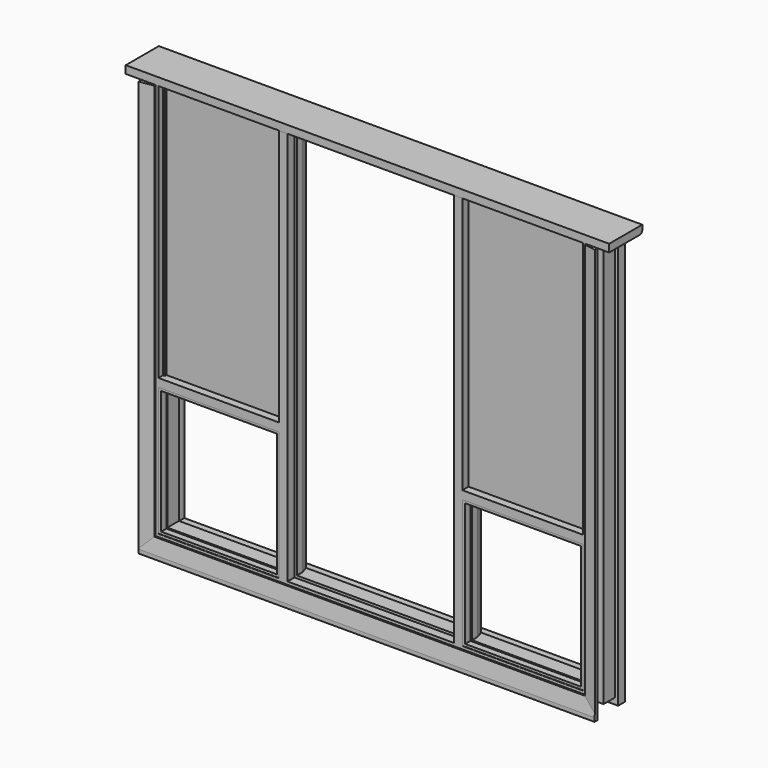
from build123d import *

# Parameters (mm, degrees)
F0_W          = 625
F0_H          = 667
F1_DEPTH      = 45
F3_W          = 645
F3_H          = 687
F3_W_2        = 599
F3_H_2        = 641
F4_DEPTH      = 34
F7_DEPTH      = 75
F9_DEPTH      = 20
F10_T1_DEPTH  = 2228
F10_T3_DEPTH  = 2249.90940659
F10_T9_DEPTH  = 2249.90940659
F10_T15_DEPTH = 2422.90940659
F10_T23_DEPTH = 2422.90940659
F10_T28_DEPTH = 2249.90940659
F11_SIZE2     = 40
F11_SIZE      = 12.5
F13_DEPTH     = 10
F15_DEPTH     = 620
F16_W         = 45
F16_H         = 1126
F17_DEPTH     = 15
F18_T4_DEPTH  = 1160.9259151598
F18_T10_DEPTH = 1160.9259151598
F18_T16_DEPTH = 1160.9259151598
F18_T22_DEPTH = 1160.9259151598
F20_DEPTH     = 44
F22_DEPTH     = 40
F23_R         = 15


# Not quite as in the source:
# - a fillet or chamfer that OpenCascade refuses, or shapes differently, is made with other operations: its cross-section is extruded or revolved along the edge and cut away or added
# - a pattern or mirror of a feature is missing from the dataset's text; its kind, count and spacing are read off the source's solid


with BuildPart() as f1:
    # F0 (on Front) → F1 (new body)
    with BuildSketch(Plane.XZ):
        Polygon((474, 0), (431, 0), (431, -2040), (-431, -2040), (-431, 0), (-474, 0), (-474, -1330), (-1099, -1330), (-1099, 0), (-1124, 0), (-1124, -2065), (1124, -2065), (1124, 0), (1099, 0), (1099, -1330), (474, -1330), align=None)
        with Locations((-786.5, -1706.5)):
            Rectangle(F0_W, F0_H, mode=Mode.SUBTRACT)
        with Locations((786.5, -1706.5)):
            Rectangle(F0_W, F0_H, mode=Mode.SUBTRACT)
    extrude(amount=F1_DEPTH)

    # F3 (on offset) → F4 (join)
    with BuildSketch(Plane.XZ.offset(43)):
        with Locations((786.5, -1706.5)):
            Rectangle(F3_W, F3_H)
        with Locations((786.5, -1706.5)):
            Rectangle(F3_W_2, F3_H_2, mode=Mode.SUBTRACT)
    extrude(amount=-F4_DEPTH)

    # F6: F1 across plane


with BuildPart() as f1_1:
    add(f1.part)
    add(f1.part.mirror(Plane.YZ))

    # F5 (on face) → F7 (join)
    with BuildSketch(Plane(origin=(0, 0, 0), x_dir=(-1, 0, 0), z_dir=(0, 1, 0))):
        Polygon((-488, -2027), (-1099, -2027), (-1099, 0), (-1169, 0), (-1169, -2097), (1169, -2097), (1169, 0), (1099, 0), (1099, -2027), (488, -2027), (488, 0), (418, 0), (418, -2027), (-418, -2027), (-418, 0), (-488, 0), align=None)
    extrude(amount=F7_DEPTH)

    # F8 (on face) → F9 (join)
    with BuildSketch(Plane.XZ.offset(45)):
        Polygon((1114, 0), (1114, -2055), (-1114, -2055), (-1114, 0), (-1187, 0), (-1187, -2150), (1174, -2150), (1174, 0), align=None)
    extrude(amount=F9_DEPTH)

    # F10: chamfer of 12 x 75 on 3 edges, made by hand

    # F10_s2 → F10_t1 (cut)
    with BuildSketch(Plane.YZ.offset(-1114)):
        Polygon((-53, -2055), (-65, -2130), (-65, -2055), align=None)
    extrude(amount=F10_T1_DEPTH, mode=Mode.SUBTRACT)

    # F10_s4 → F10_t3 (cut)
    with BuildSketch(Plane.XY.offset(-2055)):
        Polygon((-1114, -53), (-1189, -65), (-1114, -65), align=None)
        Polygon((1114, -53), (1189, -65), (1114, -65), align=None)
    extrude(amount=F10_T3_DEPTH, mode=Mode.SUBTRACT)


with BuildPart() as f10_tool7:
    # F10_s8 → F10_t9 (new body)
    with BuildSketch(Plane.XY):
        Polygon((1114, -53), (1189, -65), (1114, -65), align=None)
    extrude(amount=-F10_T9_DEPTH)

    split(bisect_by=Plane.XY.offset(-2055), keep=Keep.BOTTOM)

    split(bisect_by=Plane.YZ.offset(1174), keep=Keep.BOTTOM)

    split(bisect_by=Plane.XY.offset(-2150), keep=Keep.TOP)


with BuildPart() as f10_tool13:
    # F10_s14 → F10_t15 (new body)
    with BuildSketch(Plane.YZ.offset(1308.90940659)):
        Polygon((-53, -2055), (-65, -2130), (-65, -2055), align=None)
    extrude(amount=-F10_T15_DEPTH)

    split(bisect_by=Plane.YZ.offset(1114), keep=Keep.TOP)

    split(bisect_by=Plane.YZ.offset(1174), keep=Keep.BOTTOM)


with BuildPart() as f10_tool7_1:
    add(f10_tool7.part)

    # F10_t18: intersect F10_tool13
    add(f10_tool13.part, mode=Mode.INTERSECT)


with BuildPart() as f1_2:
    add(f1_1.part)

    # F10_t5: cut F10_tool7
    add(f10_tool7_1.part, mode=Mode.SUBTRACT)


with BuildPart() as f10_tool21:
    # F10_s22 → F10_t23 (new body)
    with BuildSketch(Plane.YZ.offset(1114)):
        Polygon((-53, -2055), (-65, -2130), (-65, -2055), align=None)
    extrude(amount=-F10_T23_DEPTH)

    split(bisect_by=Plane.YZ.offset(-1114), keep=Keep.BOTTOM)

    split(bisect_by=Plane.YZ.offset(-1187), keep=Keep.TOP)


with BuildPart() as f10_tool26:
    # F10_s27 → F10_t28 (new body)
    with BuildSketch(Plane.XY.offset(-2249.90940659)):
        Polygon((-1114, -53), (-1189, -65), (-1114, -65), align=None)
    extrude(amount=F10_T28_DEPTH)

    split(bisect_by=Plane.XY.offset(-2055), keep=Keep.BOTTOM)

    split(bisect_by=Plane.YZ.offset(-1187), keep=Keep.TOP)

    split(bisect_by=Plane.XY.offset(-2150), keep=Keep.TOP)


with BuildPart() as f10_tool21_1:
    add(f10_tool21.part)

    # F10_t32: intersect F10_tool26
    add(f10_tool26.part, mode=Mode.INTERSECT)


with BuildPart() as f1_3:
    add(f1_2.part)

    # F10_t19: cut F10_tool21
    add(f10_tool21_1.part, mode=Mode.SUBTRACT)

    # F11
    f11_edges = [f1_3.edges().sort_by_distance(p)[0] for p in [
        (-488, 75, -1013.5),
        (-418, 75, -1013.5),
        (488, 75, -1013.5),
        (418, 75, -1013.5),
    ]]
    f11_side = f1_3.faces().sort_by_distance((793.5, 75, -2058.406453))[0]
    chamfer(f11_edges, length=F11_SIZE, length2=F11_SIZE2, reference=f11_side)

    # F12 (on face) → F13 (join)
    with BuildSketch(Plane(origin=(1099, 0, 0), x_dir=(0, -1, 0), z_dir=(-1, 0, 0))):
        Polygon((0, -2027), (0, -1373), (0, -1330), (15, -1330), (15, 0), (-75, 0), (-75, -2027), align=None)
    f13 = extrude(amount=F13_DEPTH)

    # F13_copies: F13 across plane
    add(f13.mirror(Plane(origin=(0, 0, 0), x_dir=(0, 0, -1), z_dir=(-1, 0, 0))))

    # F14 (on face) → F15 (join)
    with BuildSketch(Plane(origin=(1089, 0, 0), x_dir=(0, -1, 0), z_dir=(-1, 0, 0))):
        Polygon((0, -1386), (0, -1373), (0, -1330), (5, -1330), (5, 0), (-25, 0), (-25, -190), (0, -200), (0, -1316), (-50, -1316), (-50, -1371), align=None)
    f15 = extrude(amount=F15_DEPTH)

    # F15_copies: F15 across plane
    add(f15.mirror(Plane(origin=(0, 0, 0), x_dir=(0, 0, -1), z_dir=(-1, 0, 0))))

    # F16 (on face) → F17 (join)
    with BuildSketch(Plane(origin=(0, 0, 0), x_dir=(-1, 0, 0), z_dir=(0, 1, 0))):
        with Locations((-788.5, -753)):
            Rectangle(F16_W, F16_H)
    f17 = extrude(amount=F17_DEPTH)

    # F17_copies: F17 across plane
    add(f17.mirror(Plane(origin=(0, 0, 0), x_dir=(0, 0, -1), z_dir=(-1, 0, 0))))

    # F18: chamfer of 5 x 15 on 4 edges, made by hand


with BuildPart() as f18_tool2:
    # F18_s3 → F18_t4 (new body)
    with BuildSketch(Plane.XY.offset(-1316)):
        Polygon((766, 0), (771, 15), (766, 15), align=None)
    extrude(amount=F18_T4_DEPTH)

    split(bisect_by=Plane(origin=(0, 68.9655172414, -172.4137931034), x_dir=(1, 0, 0), z_dir=(0, 0.3713906764, -0.9284766909)), keep=Keep.TOP)

    split(bisect_by=Plane.XZ, keep=Keep.BOTTOM)


with BuildPart() as f1_4:
    add(f1_3.part)

    # F18_t1: cut F18_tool2
    add(f18_tool2.part, mode=Mode.SUBTRACT)


with BuildPart() as f18_tool8:
    # F18_s9 → F18_t10 (new body)
    with BuildSketch(Plane.XY.offset(-155.0740848402)):
        Polygon((806, 15), (811, 0), (811, 15), align=None)
    extrude(amount=-F18_T10_DEPTH)

    split(bisect_by=Plane(origin=(0, 68.9655172414, -172.4137931034), x_dir=(1, 0, 0), z_dir=(0, 0.3713906764, -0.9284766909)), keep=Keep.TOP)

    split(bisect_by=Plane.XZ, keep=Keep.BOTTOM)


with BuildPart() as f1_5:
    add(f1_4.part)

    # F18_t7: cut F18_tool8
    add(f18_tool8.part, mode=Mode.SUBTRACT)


with BuildPart() as f18_tool14:
    # F18_s15 → F18_t16 (new body)
    with BuildSketch(Plane.XY.offset(-155.0740848402)):
        Polygon((-811, 0), (-806, 15), (-811, 15), align=None)
    extrude(amount=-F18_T16_DEPTH)

    split(bisect_by=Plane(origin=(0, 68.9655172414, -172.4137931034), x_dir=(1, 0, 0), z_dir=(0, 0.3713906764, -0.9284766909)), keep=Keep.TOP)

    split(bisect_by=Plane.XZ, keep=Keep.BOTTOM)


with BuildPart() as f1_6:
    add(f1_5.part)

    # F18_t13: cut F18_tool14
    add(f18_tool14.part, mode=Mode.SUBTRACT)


with BuildPart() as f18_tool20:
    # F18_s21 → F18_t22 (new body)
    with BuildSketch(Plane.XY.offset(-1316)):
        Polygon((-771, 15), (-766, 0), (-766, 15), align=None)
    extrude(amount=F18_T22_DEPTH)

    split(bisect_by=Plane(origin=(0, 68.9655172414, -172.4137931034), x_dir=(1, 0, 0), z_dir=(0, 0.3713906764, -0.9284766909)), keep=Keep.TOP)

    split(bisect_by=Plane.XZ, keep=Keep.BOTTOM)


with BuildPart() as f1_7:
    add(f1_6.part)

    # F18_t19: cut F18_tool20
    add(f18_tool20.part, mode=Mode.SUBTRACT)

    # F19 (on face) → F20 (join)
    with BuildSketch(Plane(origin=(0, 75, 0), x_dir=(-1, 0, 0), z_dir=(0, 1, 0))):
        Polygon((1096, 0), (1096, -2034), (-1096, -2034), (-1096, 0), (-1184, 0), (-1184, -2130), (1218, -2130), (1218, 0), align=None)
    extrude(amount=F20_DEPTH)


with BuildPart() as f22:
    # F21 (on face) → F22 (new body)
    with BuildSketch(Plane.XY):
        Polygon((-1268, -45), (1124, -45), (1234, -45), (1234, 169), (-1268, 169), align=None)
    extrude(amount=F22_DEPTH)

    # F23
    f23_edges = [f22.edges().sort_by_distance(p)[0] for p in [
        (-17, 169, 0),
    ]]
    fillet(f23_edges, radius=F23_R)


solid = Compound([f1_7.part, f22.part])
